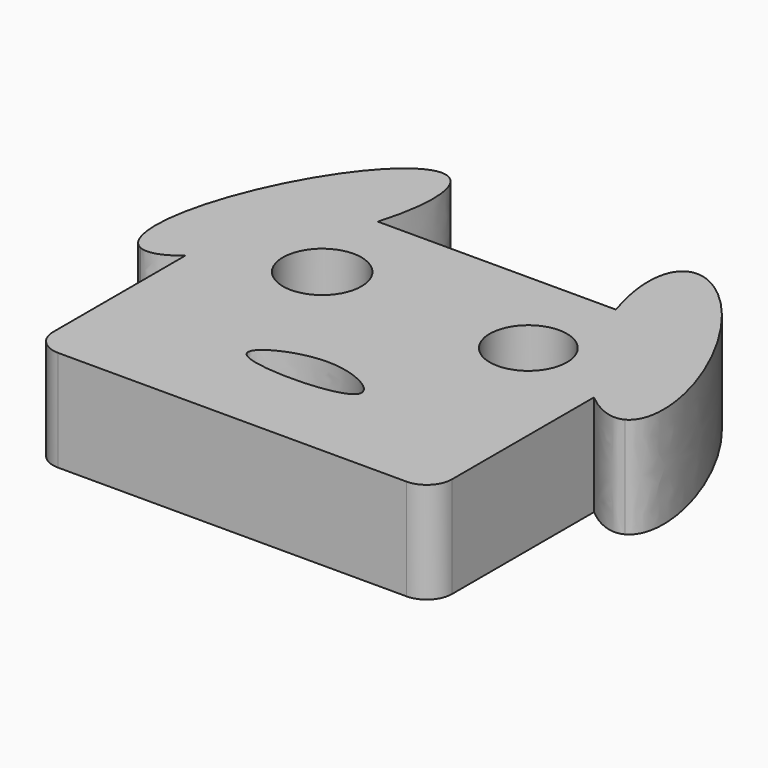
from build123d import *

# Parameters (mm, degrees)
F0_R     = 9.8728089089
F0_R_2   = 9.7111986955
F2_DEPTH = 25.4
F4_DEPTH = 25.4


# Not quite as in the source:
# - a feature of the source that left no trace in its solid (it failed there, or was rolled back) is left out


with BuildPart() as f2:
    # F0 (on Top) → F2 (new body)
    with BuildSketch(Plane.XY):
        with BuildLine():
            Line((49.9262437224, 52.69991979), (-50.352960825, 52.69991979))
            Line((-50.352960825, 52.69991979), (-50.352960825, -23.7337587565))
            ThreePointArc((-50.352960825, -23.7337587565), (-48.4930888855, -28.2238868171), (-44.002960825, -30.0837587565))
            Line((-44.002960825, -30.0837587565), (43.5762437224, -30.0837587565))
            ThreePointArc((43.5762437224, -30.0837587565), (48.066371783, -28.2238868171), (49.9262437224, -23.7337587565))
            Line((49.9262437224, -23.7337587565), (49.9262437224, 52.69991979))
        make_face()
        with BuildLine():
            add(Edge.make_bspline(
                [(-14.7778214887, -7.4204108678), (-17.0474622449, -4.724920884), (0.0101588176, 4.661771469), (24.9215305111, -10.7341156747), (-11.8554777737, -10.8910694692), (-14.7778214887, -7.4204108678)],
                knots=[0, 0, 0, 0, 0.310030383, 0.6008111246, 1, 1, 1, 1], degree=3))
        make_face(mode=Mode.SUBTRACT)
        with Locations((-25.0580441207, 29.2028859258)):
            Circle(F0_R, mode=Mode.SUBTRACT)
        with Locations((26.771415025, 29.2028859258)):
            Circle(F0_R_2, mode=Mode.SUBTRACT)
    extrude(amount=F2_DEPTH)

    # F1 (on face) → F4 (join)
    with BuildSketch(Plane.XY):
        with BuildLine():
            add(Edge.make_bspline(
                [(-29.878199615, 52.69991979), (-13.1223447166, 109.563974095), (-46.3737055212, 66.904188779), (-79.6250663257, 24.2444034629), (-59.3140795827, 14.9352001026)],
                knots=[1.9591551893, 1.9591551893, 1.9591551893, 4.1211702482, 4.1211702482, 6.2831853072, 6.2831853072, 6.2831853072], degree=2, weights=[1, 0.4704395266, 1, 0.4704395266, 1]))
            add(Edge.make_bspline(
                [(-59.3140795827, 14.9352001026), (-55.828433528, 13.3376121383), (-50.352960825, 17.8096105923)],
                knots=[0, 0, 0, 0.6228628932, 0.6228628932, 0.6228628932], degree=2, weights=[1, 0.9518959192, 1]))
            Line((-50.352960825, 17.8096105923), (-50.352960825, 52.69991979))
            Line((-50.352960825, 52.69991979), (-29.878199615, 52.69991979))
        make_face()
        with BuildLine():
            add(Edge.make_bspline(
                [(60.5942457914, 17.282159999), (79.4357554833, 27.198748734), (46.3404123224, 65.5008495201), (13.2450691614, 103.8029503062), (29.9911485665, 52.69991979)],
                knots=[0, 0, 0, 2.1384468293, 2.1384468293, 4.2768936586, 4.2768936586, 4.2768936586], degree=2, weights=[1, 0.4808053052, 1, 0.4808053052, 1]))
            Line((29.9911485665, 52.69991979), (49.9262437224, 52.69991979))
            Line((49.9262437224, 52.69991979), (49.9262437224, 20.8637133092))
            add(Edge.make_bspline(
                [(49.9262437224, 20.8637133092), (56.655587103, 15.2091807623), (60.5942457914, 17.282159999)],
                knots=[5.5547572315, 5.5547572315, 5.5547572315, 6.2831853072, 6.2831853072, 6.2831853072], degree=2, weights=[1, 0.9344040212, 1]))
        make_face()
    extrude(amount=F4_DEPTH)


solid = f2.part
